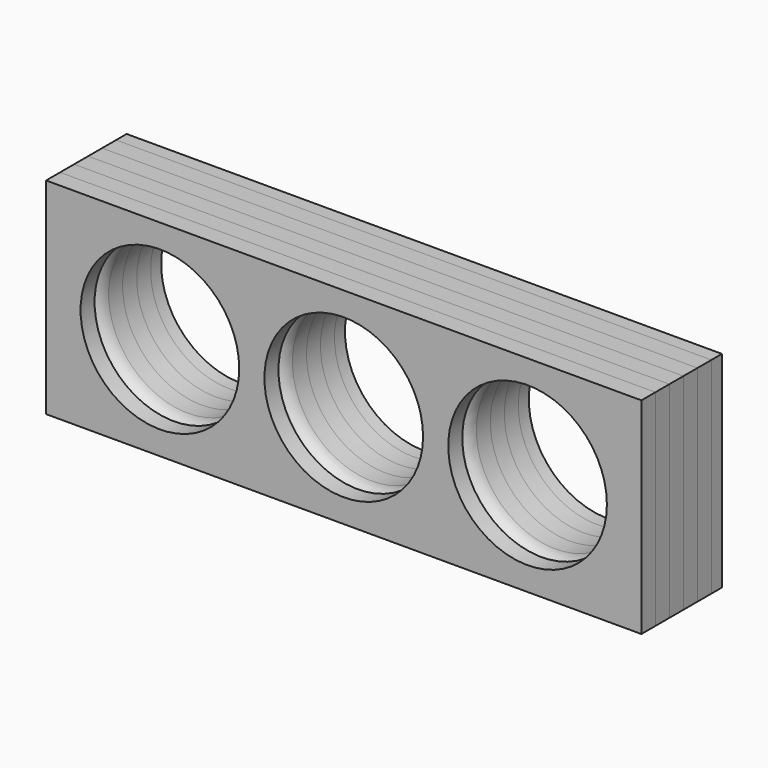
from build123d import *

# Parameters (mm, degrees)
F0_W     = 863.6
F0_H     = 298.45
F0_R     = 115.062
F1_DEPTH = 25.4
F2_DEPTH = 25.4
F3_DEPTH = 25.4
F4_DEPTH = 25.4
F5_DEPTH = 25.4
F6_DEPTH = 19.05


# Not quite as in the source:
# - a fillet or chamfer that OpenCascade refuses, or shapes differently, is made with other operations: its cross-section is extruded or revolved along the edge and cut away or added


with BuildPart() as f1:
    # F0 (on Front) → F1 (new body)
    with BuildSketch(Plane.XZ):
        Rectangle(F0_W, F0_H)
        with Locations((-266.7, 0)):
            Circle(F0_R, mode=Mode.SUBTRACT)
        Circle(F0_R, mode=Mode.SUBTRACT)
        with Locations((266.7, 0)):
            Circle(F0_R, mode=Mode.SUBTRACT)
    extrude(amount=F1_DEPTH)


with BuildPart() as f2:
    # F2 (new): a face of the model
    f2_faces = [f1.part.faces().sort_by_distance(p)[0] for p in [
        (422.6628376259, 0, 0),
    ]]
    extrude(f2_faces, amount=F2_DEPTH)


with BuildPart() as f3:
    # F3 (new): a face of the model
    f3_faces = [f2.part.faces().sort_by_distance(p)[0] for p in [
        (422.6628376259, 25.4, 0),
    ]]
    extrude(f3_faces, amount=F3_DEPTH)


with BuildPart() as f4:
    # F4 (new): a face of the model
    f4_faces = [f3.part.faces().sort_by_distance(p)[0] for p in [
        (422.6628376259, 50.8, 0),
    ]]
    extrude(f4_faces, amount=F4_DEPTH)


with BuildPart() as f5:
    # F5 (new): a face of the model
    f5_faces = [f4.part.faces().sort_by_distance(p)[0] for p in [
        (422.6628376259, 76.2, 0),
    ]]
    extrude(f5_faces, amount=F5_DEPTH)


with BuildPart() as f6:
    # F6 (new): a face of the model
    f6_faces = [f5.part.faces().sort_by_distance(p)[0] for p in [
        (422.6628376259, 101.6, 0),
    ]]
    extrude(f6_faces, amount=F6_DEPTH)


with BuildPart() as f2_1:
    add(f2.part)

    # F7: fillet of radius 25.4 on 3 edges, made by hand

    # F7_s1 → F7_t2 (revolve, cut)
    with BuildSketch(Plane.XY):
        with BuildLine():
            ThreePointArc((-151.638, 25.4), (-144.1985122421, 7.4394877579), (-126.238, 0))
            Line((-126.238, 0), (-151.638, 0))
            Line((-151.638, 0), (-151.638, 25.4))
        make_face()
    revolve(axis=Axis((-266.7, 0, 0), (0, -1, 0)), mode=Mode.SUBTRACT)

    # F7_s3 → F7_t4 (revolve, cut)
    with BuildSketch(Plane.XY):
        with BuildLine():
            ThreePointArc((115.062, 25.4), (122.5014877579, 7.4394877579), (140.462, 0))
            Line((140.462, 0), (115.062, 0))
            Line((115.062, 0), (115.062, 25.4))
        make_face()
    revolve(axis=Axis((0, 0, 0), (0, -1, 0)), mode=Mode.SUBTRACT)

    # F7_s5 → F7_t6 (revolve, cut)
    with BuildSketch(Plane.XY):
        with BuildLine():
            ThreePointArc((381.762, 25.4), (389.2014877579, 7.4394877579), (407.162, 0))
            Line((407.162, 0), (381.762, 0))
            Line((381.762, 0), (381.762, 25.4))
        make_face()
    revolve(axis=Axis((266.7, 0, 0), (0, -1, 0)), mode=Mode.SUBTRACT)


solid = Compound([f1.part, f3.part, f4.part, f5.part, f6.part, f2_1.part])
